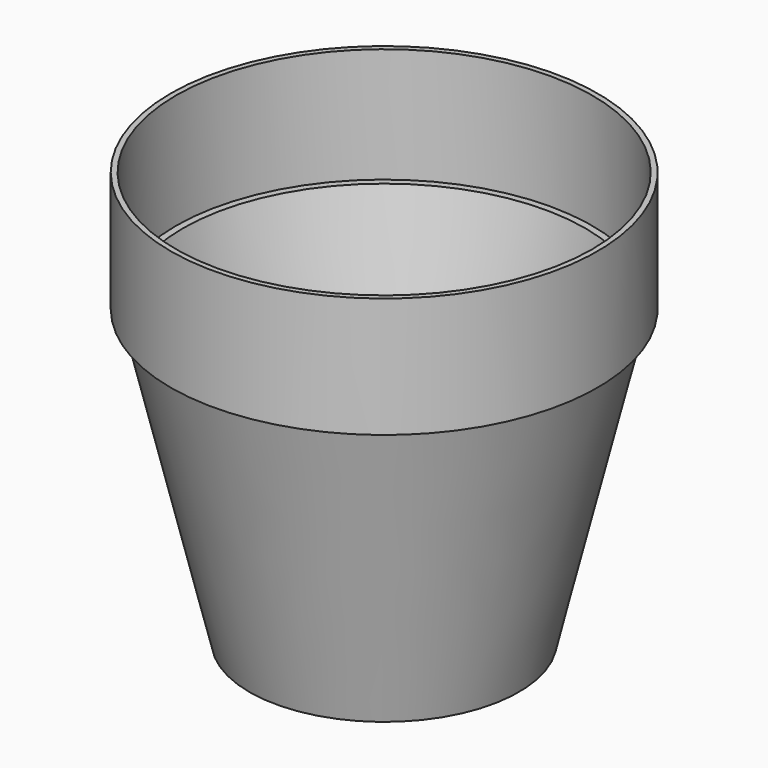
from build123d import *

# Parameters (mm, degrees)
F2_T = -2


# Not quite as in the source:
# - a feature names something its author has since deleted; it is built from what else it names


with BuildPart() as f1:
    # F0 (on Front) → F1 (revolve)
    with BuildSketch(Plane.XZ):
        Polygon((0, -91.5846474071), (0, 63.4153525929), (-80, 63.4153525929), (-80, 18.4153525929), (-77, 18.4153525929), (-50.5, -91.5846474071), align=None)
    revolve(axis=Axis((0, 0, -14.0846474071), (0, 0, -1)))

    # F2
    f2_openings = [f1.faces().sort_by_distance(p)[0] for p in [
        (0, 0, 63.415353),
    ]]
    offset(amount=F2_T, openings=f2_openings, kind=Kind.INTERSECTION)


solid = f1.part
